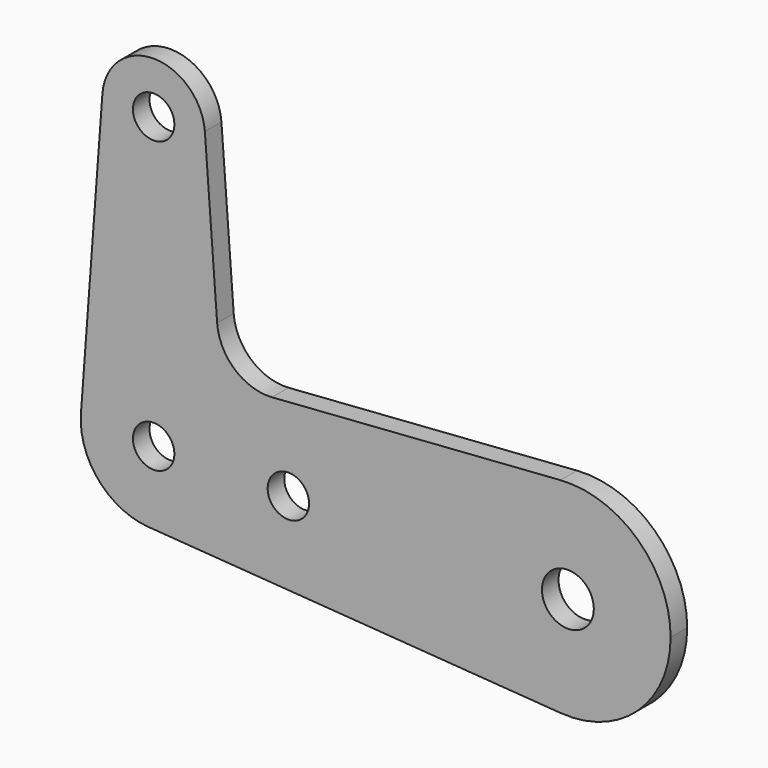
from build123d import *

# Parameters (mm, degrees)
F1_DEPTH = 3.175
F2_R     = 3.9751
F2_R_2   = 3.175
F3_DEPTH = 3.176


with BuildPart() as f1:
    # F0 (on Front) → F1 (new body)
    with BuildSketch(Plane.XZ):
        with BuildLine():
            ThreePointArc((-1.133856, -15.7071281452), (10.7271510596, -11.5294290467), (15.748, 0))
            ThreePointArc((15.748, 0), (10.7271378512, 11.529441336), (-1.1338919889, 15.7071255473))
            ThreePointArc((-1.1338919889, 15.7071255473), (-11.529441336, 10.7271378512), (-15.748, 0))
            ThreePointArc((-15.748, 0), (-11.5294290467, -10.7271510596), (-1.133856, -15.7071281452))
        make_face()
        with BuildLine():
            ThreePointArc((-15.748, 0), (-11.529441336, 10.7271378512), (-1.1338919889, 15.7071255473))
            Line((-1.1338919889, 15.7071255473), (-45.34766523, 12.5153484696))
            ThreePointArc((-45.34766523, 12.5153484696), (-51.0602172111, 14.4088260903), (-53.7668572171, 19.7840105071))
            Line((-53.7668572171, 19.7840105071), (-55.6477540074, 45.0349007362))
            ThreePointArc((-55.6477540074, 45.0349007362), (-55.6314403813, 44.7426525705), (-55.626, 44.45))
            ThreePointArc((-55.626, 44.45), (-57.9322412049, 38.8822412049), (-63.5, 36.576))
            ThreePointArc((-63.5, 36.576), (-69.270857002, 39.0930339311), (-71.352244132, 45.0349257143))
            Line((-71.352244132, 45.0349257143), (-74.6451207035, 0.8302171429))
            ThreePointArc((-74.6451207035, 0.8302171429), (-63.0846043948, 11.1682775078), (-52.324, 0))
            ThreePointArc((-52.324, 0), (-55.887183119, -8.1821754525), (-64.304672, -11.1469941676))
            Line((-64.304672, -11.1469941676), (-1.133856, -15.7071281452))
            ThreePointArc((-1.133856, -15.7071281452), (-11.5294290467, -10.7271510596), (-15.748, 0))
        make_face()
        with BuildLine():
            ThreePointArc((-74.6451207035, 0.8302171429), (-71.9594789501, -7.3034369917), (-64.304672, -11.1469941676))
            ThreePointArc((-64.304672, -11.1469941676), (-55.887183119, -8.1821754525), (-52.324, 0))
            ThreePointArc((-52.324, 0), (-63.0846043948, 11.1682775078), (-74.6451207035, 0.8302171429))
        make_face()
        with BuildLine():
            ThreePointArc((-55.626, 44.45), (-55.6314403813, 44.7426525705), (-55.6477540074, 45.0349007362))
            ThreePointArc((-55.6477540074, 45.0349007362), (-63.4999874763, 52.324), (-71.352244132, 45.0349257143))
            ThreePointArc((-71.352244132, 45.0349257143), (-69.270857002, 39.0930339311), (-63.5, 36.576))
            ThreePointArc((-63.5, 36.576), (-57.9322412049, 38.8822412049), (-55.626, 44.45))
        make_face()
    extrude(amount=F1_DEPTH)

    # F2 (on face) → F3 (cut, through all)
    with BuildSketch(Plane.XZ.offset(3.175)):
        Circle(F2_R)
        with Locations((-63.5, 0)):
            Circle(F2_R_2)
        with Locations((-42.8498, 0)):
            Circle(F2_R_2)
        with Locations((-63.5, 44.45)):
            Circle(F2_R_2)
    extrude(amount=-F3_DEPTH, mode=Mode.SUBTRACT)


solid = f1.part
